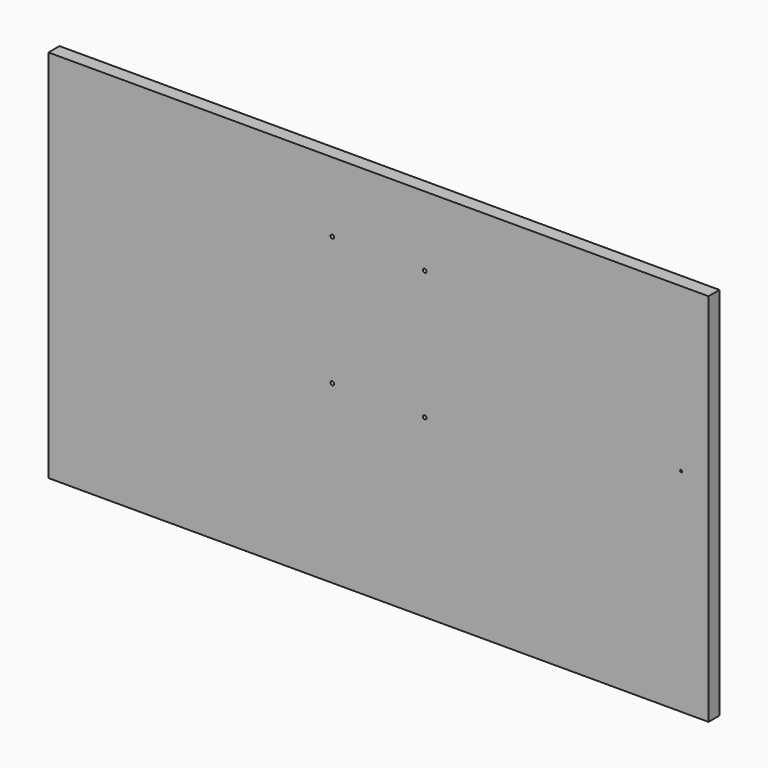
from build123d import *

# Parameters (mm, degrees)
F0_W     = 914.4
F0_H     = 519.176
F1_DEPTH = 19.05
F3_D     = 5.0038
F3_DEPTH = 25.4
F3_TIP   = 1.5032931827
F5_D     = 3.175
F5_DEPTH = 14.224
F5_TIP   = 0.9538662327


with BuildPart() as f1:
    # F0 (on Front) → F1 (new body)
    with BuildSketch(Plane.XZ):
        Rectangle(F0_W, F0_H)
    extrude(amount=F1_DEPTH)

    # F3
    with Locations(Plane.XZ.offset(19.05)):
        with Locations((-64.008, 162.814), (64.008, 162.814), (-64.008, -16.002), (64.008, -16.002)):
            Hole(F3_D / 2, depth=F3_DEPTH)
            with Locations((0, 0, -(F3_DEPTH + F3_TIP / 2))):  # 118° drill point
                Cone(0, F3_D / 2, F3_TIP, mode=Mode.SUBTRACT)

    # F5
    with Locations(Plane.XZ.offset(19.05)):
        with Locations((419.1, 34.036)):
            Hole(F5_D / 2, depth=F5_DEPTH)
            with Locations((0, 0, -(F5_DEPTH + F5_TIP / 2))):  # 118° drill point
                Cone(0, F5_D / 2, F5_TIP, mode=Mode.SUBTRACT)


solid = f1.part
